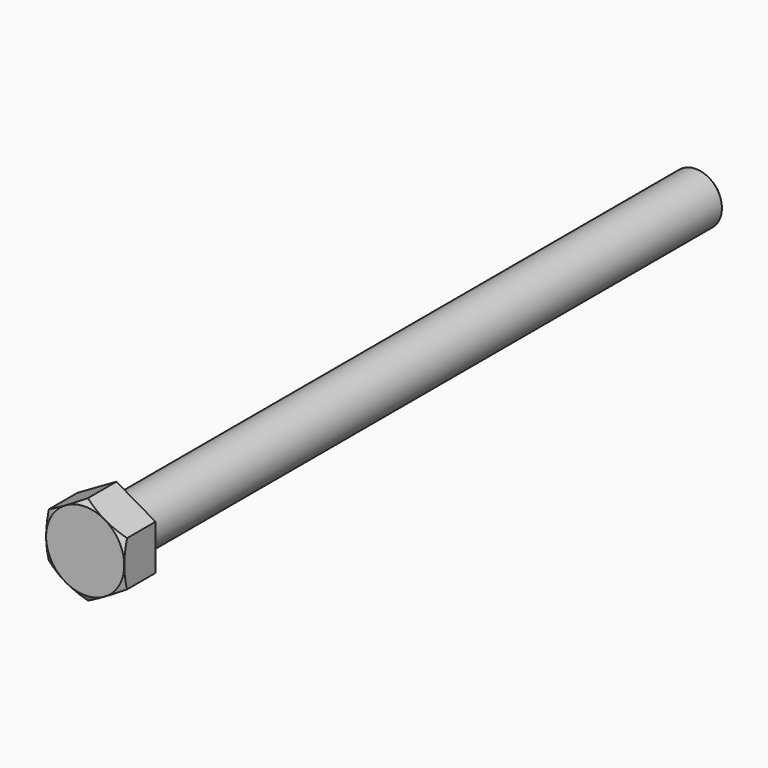
from build123d import *

# Parameters (mm, degrees)
F2_R     = 3.175
F3_DEPTH = 88.9
F5_DEPTH = 4.7625
F6_SIZE  = 0.635


# Not quite as in the source:
# - a length typed as a fraction of an inch, garbled in the dataset ("3 / 203.2 mm" for 3/8 in), is restored


with BuildPart() as f3:
    # F2 (on Front) → F3 (new body)
    with BuildSketch(Plane.XZ):
        Circle(F2_R)
    extrude(amount=-F3_DEPTH)

    # F4 (on Front) → F5 (join)
    with BuildSketch(Plane.XZ):
        Polygon((0, -5.499261314), (4.7625, -2.749630657), (4.7625, 2.749630657), (0, 5.499261314), (-4.7625, 2.749630657), (-4.7625, -2.749630657), align=None)
    extrude(amount=F5_DEPTH)

    # F6
    f6_edges = [f3.edges().sort_by_distance(p)[0] for p in [
        (-3.175, 88.9, 0),
    ]]
    chamfer(f6_edges, length=F6_SIZE)

    # F7 (on Top) → F8 (revolve, cut)
    with BuildSketch(Plane.XY):
        Polygon((11.8464599431, -4.7625), (11.8464599431, -0.6725738199), (4.7625, -4.7625), align=None)
    revolve(axis=Axis((0, -2.38125, 0), (0, -1, 0)), mode=Mode.SUBTRACT)


solid = f3.part
